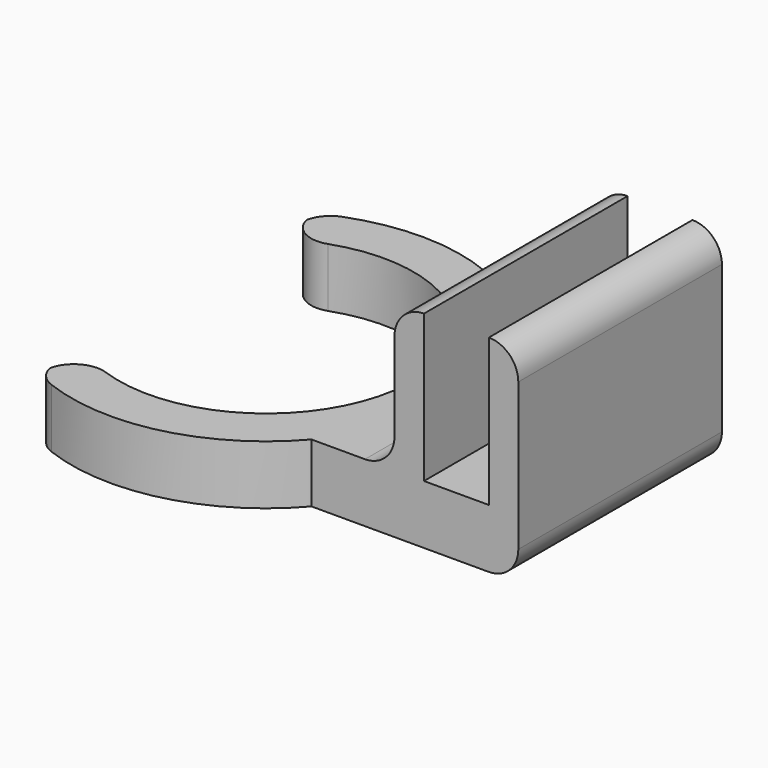
from build123d import *

# Parameters (mm, degrees)
F0_W          = 5
F0_H          = 43.1665030722
F0_W_2        = 11
F1_DEPTH      = 5
F1_DEPTH_BACK = 5
F2_T1_DEPTH   = 51.4213562373
F2_T3_DEPTH   = 27.589671948
F3_W          = 5
F3_H          = 43.1665030722
F4_DEPTH      = 25
F5_R          = 4.99999


# Not quite as in the source:
# - a fillet or chamfer that OpenCascade refuses, or shapes differently, is made with other operations: its cross-section is extruded or revolved along the edge and cut away or added
# - a fillet or chamfer is up to 0.001 mm smaller than in the source, because OpenCascade refuses the exact size
# - a feature names something its author has since deleted; it is built from what else it names


with BuildPart() as f1:
    # F0 (on Top) → F1 (new body, two sides)
    with BuildSketch(Plane.XY) as f1_sk:
        with BuildLine():
            ThreePointArc((-7.0367619663, -1.3552663468), (-21.4300874517, -22.6556162733), (-47, -20))
            Line((-47, -20), (-47, -29.3938769134))
            ThreePointArc((-47, -29.3938769134), (-25.6700714676, -32.3872197753), (-7.0367619663, -21.5832515361))
            Line((-7.0367619663, -21.5832515361), (-7.0367619663, -1.3552663468))
        make_face()
        with BuildLine():
            Line((-7.0367619663, 1.3552663468), (-7.0367619663, -1.3552663468))
            ThreePointArc((-7.0367619663, -1.3552663468), (-7, 0), (-7.0367619663, 1.3552663468))
        make_face()
        with BuildLine():
            ThreePointArc((-7.0367619663, 1.3552663468), (-7, 0), (-7.0367619663, -1.3552663468))
            Line((-7.0367619663, -1.3552663468), (-7.0367619663, -21.5832515361))
            ThreePointArc((-7.0367619663, -21.5832515361), (1, 0), (-7.0367619663, 21.5832515361))
            Line((-7.0367619663, 21.5832515361), (-7.0367619663, 1.3552663468))
        make_face()
        with BuildLine():
            ThreePointArc((-47, 20), (-21.4300874517, 22.6556162733), (-7.0367619663, 1.3552663468))
            Line((-7.0367619663, 1.3552663468), (-7.0367619663, 21.5832515361))
            ThreePointArc((-7.0367619663, 21.5832515361), (-25.6700714676, 32.3872197753), (-47, 29.3938769134))
            Line((-47, 29.3938769134), (-47, 20))
        make_face()
        with BuildLine():
            ThreePointArc((-7.0367619663, 21.5832515361), (1, 0), (-7.0367619663, -21.5832515361))
            Line((-7.0367619663, -21.5832515361), (7.0367619663, -21.5832515361))
            Line((7.0367619663, -21.5832515361), (7.0367619663, 21.5832515361))
            Line((7.0367619663, 21.5832515361), (-7.0367619663, 21.5832515361))
        make_face()
        with Locations((9.5367619663, 0)):
            Rectangle(F0_W, F0_H)
        with Locations((17.5367619663, 0)):
            Rectangle(F0_W_2, F0_H)
        with Locations((25.5367619663, 0)):
            Rectangle(F0_W, F0_H)
    extrude(amount=F1_DEPTH)
    extrude(f1_sk.sketch, amount=-F1_DEPTH_BACK)

    # F2: fillet of radius 5 on 4 edges, made by hand

    # F2_s2 → F2_t1 (cut)
    with BuildSketch(Plane.XY.offset(-25.7106781187)):
        with BuildLine():
            ThreePointArc((-40.3333333333, 23.5702260396), (-44.8867513459, 24.2017883428), (-47, 28.2842712475))
            Line((-47, 28.2842712475), (-47, 20))
            ThreePointArc((-47, 20), (-43.8024463398, 22.0386537791), (-40.3333333333, 23.5702260396))
        make_face()
        with BuildLine():
            ThreePointArc((-40.3333333333, -23.5702260396), (-44.8867513459, -24.2017883428), (-47, -28.2842712475))
            Line((-47, -28.2842712475), (-47, -20))
            ThreePointArc((-47, -20), (-43.8024463398, -22.0386537791), (-40.3333333333, -23.5702260396))
        make_face()
    extrude(amount=F2_T1_DEPTH, mode=Mode.SUBTRACT)

    # F2_s4 → F2_t3 (cut)
    with BuildSketch(Plane.XY.offset(-13.794835974)):
        with BuildLine():
            ThreePointArc((-43.7857142857, -30.8236425293), (-46.1187723552, -28.9881272088), (-47, -26.1533936612))
            Line((-47, -26.1533936612), (-47, -29.3938769134))
            ThreePointArc((-47, -29.3938769134), (-45.4119230492, -30.1516221806), (-43.7857142857, -30.8236425293))
        make_face()
        with BuildLine():
            ThreePointArc((-47, 26.1533936612), (-46.1187723552, 28.9881272088), (-43.7857142857, 30.8236425293))
            ThreePointArc((-43.7857142857, 30.8236425293), (-45.4119230492, 30.1516221806), (-47, 29.3938769134))
            Line((-47, 29.3938769134), (-47, 26.1533936612))
        make_face()
    extrude(amount=F2_T3_DEPTH, mode=Mode.SUBTRACT)

    # F3 (on face) → F4 (join)
    with BuildSketch(Plane.XY.offset(5)):
        with Locations((9.5367619663, 0)):
            Rectangle(F3_W, F3_H)
        with Locations((25.5367619663, 0)):
            Rectangle(F3_W, F3_H)
    extrude(amount=F4_DEPTH)

    # F5 (radius 5 in the source; OpenCascade refuses exactly that, so slightly less here)
    f5_edges = [f1.edges().sort_by_distance(p)[0] for p in [
        (7.036762, 0, 5),
        (7.036762, 0, 30),
        (28.036762, 0, 30),
        (28.036762, 0, -5),
    ]]
    fillet(f5_edges, radius=F5_R)


solid = f1.part
